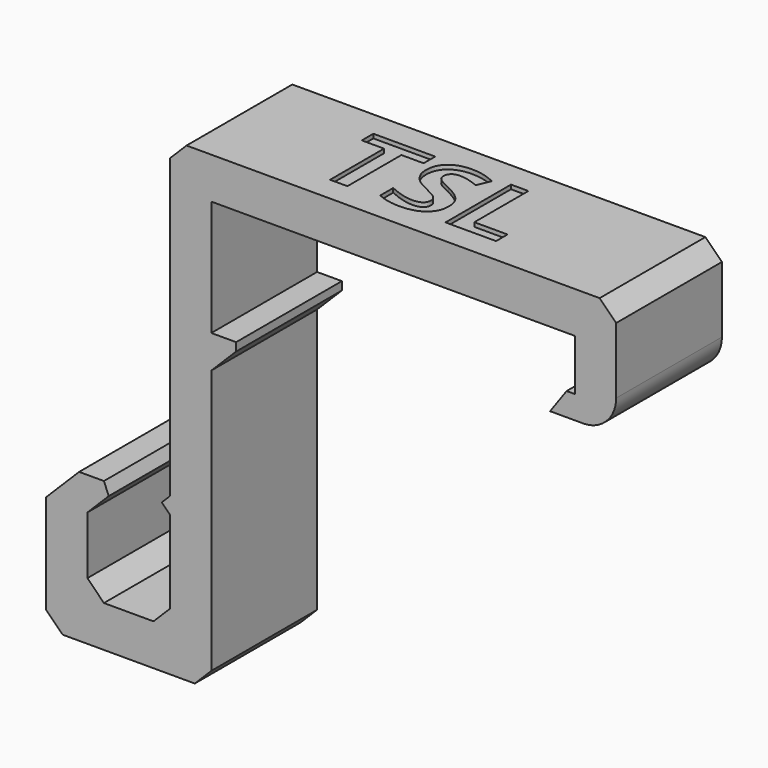
from build123d import *

# Parameters (mm, degrees)
F1_DEPTH     = 8
F2_T4_DEPTH  = 18.2867319519
F3_R         = 2
F4_SIZE      = 1
F5_TEXT_SIZE = 6.9444444444
F6_DEPTH     = 0.25
F7_SIZE      = 1


# Not quite as in the source:
# - a fillet or chamfer that OpenCascade refuses, or shapes differently, is made with other operations: its cross-section is extruded or revolved along the edge and cut away or added
# - Text() gives the source's letters only with a copy of the font that has no kerning and outlines rounded to 1/6400 em; it was checked with that copy


with BuildPart() as f1:
    # F0 (on Front) → F1 (new body)
    with BuildSketch(Plane.XZ):
        Polygon((-0.5, 18.5), (-0.5, 25.5), (21.5, 25.5), (21.5, 22.4), (21, 22.4), (20, 21), (24, 21), (24, 22.4), (24, 28), (21.5, 28), (-0.5, 28), (-3, 28), (-3, 25.5), (-3, 9), (-3.5, 8.5), (-3, 8), (-3, 2), (-8, 2), (-8, 6.5), (-6, 8.5), (-8.5, 8.5), (-10.5, 6.5), (-10.5, -0.5), (-0.5, -0.5), (-0.5, 16), (1, 16), (1, 18.5), align=None)
    extrude(amount=F1_DEPTH)

    # F2: chamfer of 2 on 1 edges, made by hand


with BuildPart() as f2_tool2:
    # F2_s3 → F2_t4 (new body)
    with BuildSketch(Plane.XZ.offset(-5.1433659759)):
        Polygon((1, 18), (-1, 16), (1, 16), align=None)
    extrude(amount=F2_T4_DEPTH)

    split(bisect_by=Plane.YZ.offset(-0.5), keep=Keep.TOP)


with BuildPart() as f1_1:
    add(f1.part)

    # F2_t1: cut F2_tool2
    add(f2_tool2.part, mode=Mode.SUBTRACT)

    # F3
    f3_edges = [f1_1.edges().sort_by_distance(p)[0] for p in [
        (24, -4, 21),
    ]]
    fillet(f3_edges, radius=F3_R)

    # F4
    f4_edges = [f1_1.edges().sort_by_distance(p)[0] for p in [
        (-0.5, -4, -0.5),
        (-3, -4, 2),
        (24, -4, 28),
        (-3, -4, 28),
        (-8, -4, 2),
        (-10.5, -4, -0.5),
    ]]
    chamfer(f4_edges, length=F4_SIZE)

    # F5 (on face) → F6 (cut)
    with BuildSketch(Plane.XY.offset(28)):
        with Locations((4, -6.5)):
            Text('TSL', F5_TEXT_SIZE, font='Open Sans', font_style=FontStyle.BOLD, text_align=(TextAlign.LEFT, TextAlign.BOTTOM))
    extrude(amount=-F6_DEPTH, mode=Mode.SUBTRACT)

    # F7
    f7_edges = [f1_1.edges().sort_by_distance(p)[0] for p in [
        (-6, -4, 8.5),
    ]]
    chamfer(f7_edges, length=F7_SIZE)


solid = f1_1.part
